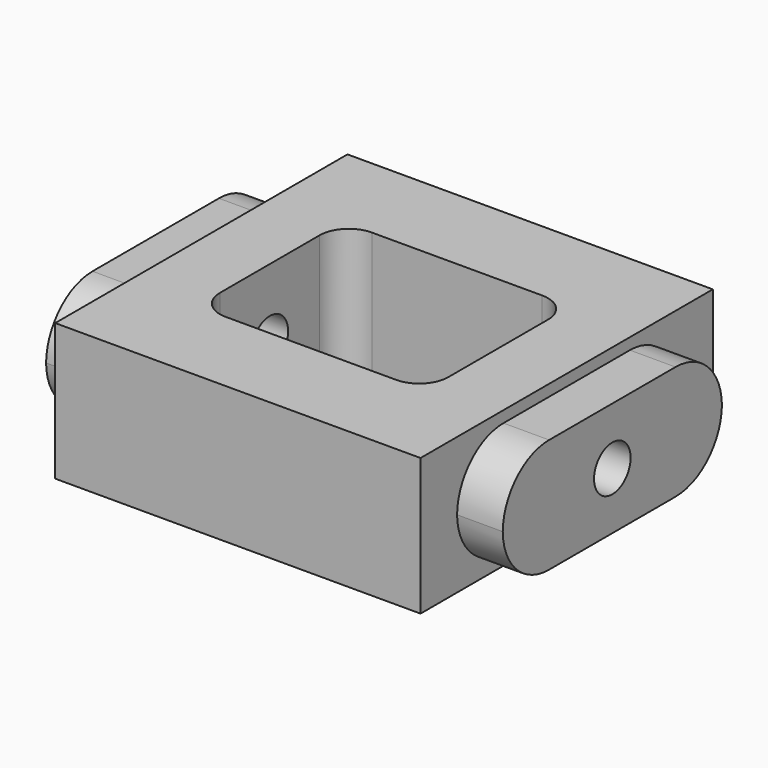
from build123d import *

# Parameters (mm, degrees)
F0_W         = 80
F0_H         = 80
F1_DEPTH     = 30
F2_W         = 60
F2_H         = 25
F3_DEPTH     = 10
F4_W         = 60
F4_H         = 25
F5_DEPTH     = 10
F6_R         = 5
F7_DEPTH     = 100.001
F8_W         = 50
F8_H         = 40
F9_DEPTH     = 30.001
F10_R        = 6.35
F11_T1_DEPTH = 41.75
F11_T3_DEPTH = 41.75


# Not quite as in the source:
# - a fillet or chamfer that OpenCascade refuses, or shapes differently, is made with other operations: its cross-section is extruded or revolved along the edge and cut away or added


with BuildPart() as f1:
    # F0 (on Top) → F1 (new body)
    with BuildSketch(Plane.XY):
        Rectangle(F0_W, F0_H)
    extrude(amount=F1_DEPTH)

    # F2 (on face) → F3 (join)
    with BuildSketch(Plane(origin=(-40, 0, 0), x_dir=(0, -1, 0), z_dir=(-1, 0, 0))):
        with Locations((0, 15)):
            Rectangle(F2_W, F2_H)
    extrude(amount=F3_DEPTH)

    # F4 (on face) → F5 (join)
    with BuildSketch(Plane.YZ.offset(40)):
        with Locations((0, 15)):
            Rectangle(F4_W, F4_H)
    extrude(amount=F5_DEPTH)

    # F6 (on face) → F7 (cut, through all)
    with BuildSketch(Plane(origin=(-50, 0, 0), x_dir=(0, -1, 0), z_dir=(-1, 0, 0))):
        with Locations((0, 15)):
            Circle(F6_R)
    extrude(amount=-F7_DEPTH, mode=Mode.SUBTRACT)

    # F8 (on face) → F9 (cut, through all)
    with BuildSketch(Plane.XY.offset(30)):
        Rectangle(F8_W, F8_H)
    extrude(amount=-F9_DEPTH, mode=Mode.SUBTRACT)

    # F10
    f10_edges = [f1.edges().sort_by_distance(p)[0] for p in [
        (-25, 20, 15),
        (25, 20, 15),
        (25, -20, 15),
        (-25, -20, 15),
    ]]
    fillet(f10_edges, radius=F10_R)

    # F11: fillet of radius 12.7 on 8 edges, made by hand

    # F11_s2 → F11_t1 (cut)
    with BuildSketch(Plane.YZ.offset(40)):
        with BuildLine():
            ThreePointArc((-30, 14.8), (-26.2802561211, 23.7802561211), (-17.3, 27.5))
            Line((-17.3, 27.5), (-30, 27.5))
            Line((-30, 27.5), (-30, 14.8))
        make_face()
        with BuildLine():
            ThreePointArc((-30, 15.2), (-26.2802561211, 6.2197438789), (-17.3, 2.5))
            Line((-17.3, 2.5), (-30, 2.5))
            Line((-30, 2.5), (-30, 15.2))
        make_face()
        with BuildLine():
            ThreePointArc((30, 15.2), (26.2802561211, 6.2197438789), (17.3, 2.5))
            Line((17.3, 2.5), (30, 2.5))
            Line((30, 2.5), (30, 15.2))
        make_face()
        with BuildLine():
            ThreePointArc((17.3, 27.5), (26.2802561211, 23.7802561211), (30, 14.8))
            Line((30, 14.8), (30, 27.5))
            Line((30, 27.5), (17.3, 27.5))
        make_face()
    extrude(amount=F11_T1_DEPTH, mode=Mode.SUBTRACT)

    # F11_s4 → F11_t3 (cut)
    with BuildSketch(Plane.YZ.offset(-81.75)):
        with BuildLine():
            ThreePointArc((17.3, 2.5), (26.2802561211, 6.2197438789), (30, 15.2))
            Line((30, 15.2), (30, 2.5))
            Line((30, 2.5), (17.3, 2.5))
        make_face()
        with BuildLine():
            ThreePointArc((-17.3, 2.5), (-26.2802561211, 6.2197438789), (-30, 15.2))
            Line((-30, 15.2), (-30, 2.5))
            Line((-30, 2.5), (-17.3, 2.5))
        make_face()
        with BuildLine():
            ThreePointArc((-17.3, 27.5), (-26.2802561211, 23.7802561211), (-30, 14.8))
            Line((-30, 14.8), (-30, 27.5))
            Line((-30, 27.5), (-17.3, 27.5))
        make_face()
        with BuildLine():
            ThreePointArc((30, 14.8), (26.2802561211, 23.7802561211), (17.3, 27.5))
            Line((17.3, 27.5), (30, 27.5))
            Line((30, 27.5), (30, 14.8))
        make_face()
    extrude(amount=F11_T3_DEPTH, mode=Mode.SUBTRACT)


solid = f1.part
